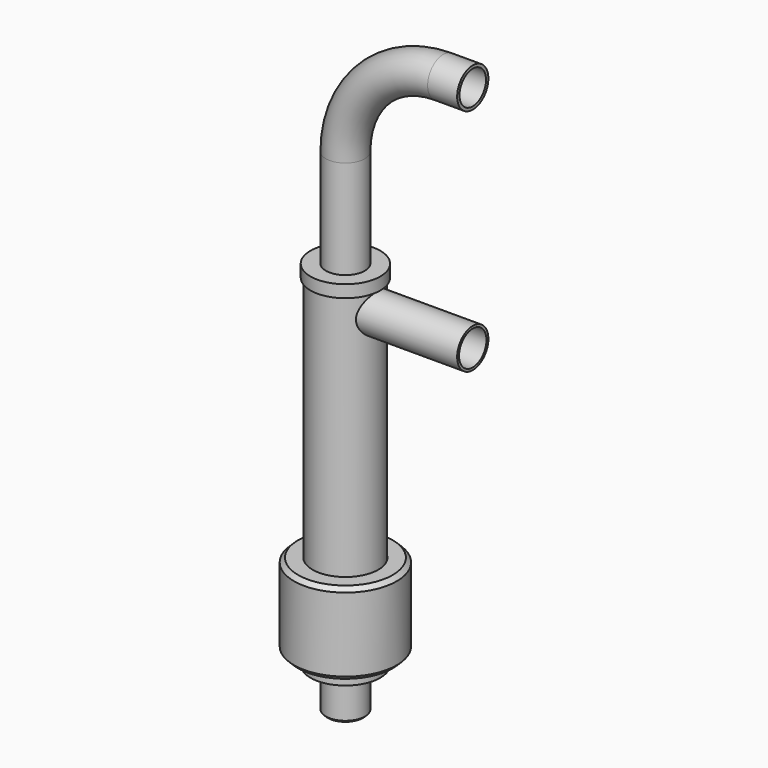
from build123d import *

# Parameters (mm, degrees)
F0_R          = 4.75
F0_R_2        = 4.0388
F1_DEPTH      = 107
F1_DEPTH_BACK = 13
F0_R_3        = 7.95
F0_R_4        = 7.2388
F2_DEPTH      = 80
F0_R_5        = 8.5
F3_DEPTH      = 3
F4_W          = 4.5
F4_H          = 20
F6_R          = 1.55
F7_DEPTH      = 12.501
F8_COUNT      = 4
F9_SIZE       = 0.5
F10_R         = 8.5
F10_R_2       = 4.75
F11_DEPTH     = 3
F12_R         = 4.75
F13_DEPTH     = 12.501
F15_R         = 4.75
F15_R_2       = 4.17088
F16_DEPTH     = 25
F18_SIZE      = 1
F1_FACE_R     = 4.75
F1_FACE_R_2   = 4.0388


with BuildPart() as f1:
    # F0 (on Top) → F1 (new body, two sides)
    with BuildSketch(Plane.XY) as f1_sk:
        Circle(F0_R)
        Circle(F0_R_2, mode=Mode.SUBTRACT)
    extrude(amount=F1_DEPTH)
    extrude(f1_sk.sketch, amount=-F1_DEPTH_BACK)

    # F9
    f9_edges = [f1.edges().sort_by_distance(p)[0] for p in [
        (-4.75, 0, -13),
    ]]
    chamfer(f9_edges, length=F9_SIZE)

    # F20: sweep along a path in F19
    with BuildLine(Plane.XZ) as f20_path:
        ThreePointArc((0, 107), (6.974519773, 123.837980227), (23.8125, 130.8125))
        Line((23.8125, 130.8125), (31, 130.8125))
    # F1_face (on face) → F20 (sweep)
    with BuildSketch(Plane.XY.offset(107)):
        Circle(F1_FACE_R)
        Circle(F1_FACE_R_2, mode=Mode.SUBTRACT)
    sweep(path=f20_path.line)


with BuildPart() as f2:
    # F0 (on Top) → F2 (new body)
    with BuildSketch(Plane.XY):
        Circle(F0_R_3)
        Circle(F0_R_4, mode=Mode.SUBTRACT)
    extrude(amount=F2_DEPTH)

    # F6 (on Front) → F7 (cut, through all)
    with BuildSketch(Plane.XZ):
        with Locations((0, 1.6)):
            Circle(F6_R)
    f7 = extrude(amount=-F7_DEPTH, mode=Mode.SUBTRACT)

    # F8: F7 ×4 about axis
    f8_axis = Axis((0, 0, 0), (0, 0, -1))
    for i in range(1, F8_COUNT):
        add(f7.rotate(f8_axis, i * 360 / F8_COUNT), mode=Mode.SUBTRACT)

    # F12 (on Right) → F13 (cut, through all)
    with BuildSketch(Plane.YZ):
        with Locations((0, 75)):
            Circle(F12_R)
    extrude(amount=F13_DEPTH, mode=Mode.SUBTRACT)


with BuildPart() as f3:
    # F0 (on Top) → F3 (new body)
    with BuildSketch(Plane.XY):
        Circle(F0_R_5)
        Circle(F0_R_3, mode=Mode.SUBTRACT)
        Circle(F0_R_3)
        Circle(F0_R_4, mode=Mode.SUBTRACT)
        Circle(F0_R_4)
        Circle(F0_R, mode=Mode.SUBTRACT)
    extrude(amount=-F3_DEPTH)


with BuildPart() as f5:
    # F4 (on Front) → F5 (revolve)
    with BuildSketch(Plane.XZ):
        with Locations((10.25, 10)):
            Rectangle(F4_W, F4_H)
    revolve(axis=Axis((0, 0, 8.3533200433), (0, 0, 1)))

    # F18
    f18_edges = [f5.edges().sort_by_distance(p)[0] for p in [
        (-12.5, 0, 0),
        (-12.5, 0, 20),
    ]]
    chamfer(f18_edges, length=F18_SIZE)


with BuildPart() as f11:
    # F10 (on face) → F11 (new body)
    with BuildSketch(Plane.XY.offset(80)):
        Circle(F10_R)
        Circle(F10_R_2, mode=Mode.SUBTRACT)
    extrude(amount=F11_DEPTH)


with BuildPart() as f16:
    # F15 (on offset) → F16 (new body)
    with BuildSketch(Plane.YZ.offset(31)):
        with Locations((0, 75)):
            Circle(F15_R)
        with Locations((0, 75)):
            Circle(F15_R_2, mode=Mode.SUBTRACT)
    extrude(amount=-F16_DEPTH)


solid = Compound([f1.part, f2.part, f3.part, f5.part, f11.part, f16.part])
